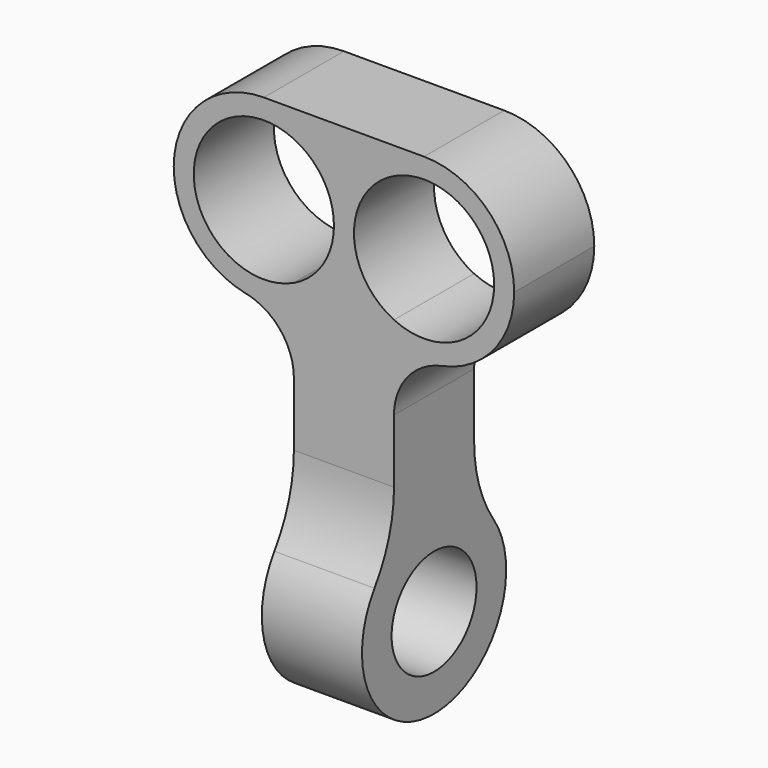
from build123d import *

# Parameters (mm, degrees)
F0_W        = 5
F0_H        = 16
F1_DEPTH    = 5
F2_R        = 4.49999
F3_T1_DEPTH = 22.5
F4_R        = 3
F5_R        = 4.5
F6_DEPTH    = 2.5
F7_R        = 2.65
F8_DEPTH    = 25
F9_R        = 7


# Not quite as in the source:
# - a fillet or chamfer that OpenCascade refuses, or shapes differently, is made with other operations: its cross-section is extruded or revolved along the edge and cut away or added
# - a fillet or chamfer is up to 0.001 mm smaller than in the source, because OpenCascade refuses the exact size


with BuildPart() as f1:
    # F0 (on Front) → F1 (new body)
    with BuildSketch(Plane.XZ):
        with BuildLine():
            Line((8.5, 12.5), (2.5, 12.5))
            Line((2.5, 12.5), (2.5, 11.1622776602))
            ThreePointArc((2.5, 11.1622776602), (5.8708286934, 10.9580398915), (7.5, 8))
            ThreePointArc((7.5, 8), (5.8708286934, 5.0419601085), (2.5, 4.8377223398))
            Line((2.5, 4.8377223398), (2.5, 3.5))
            Line((2.5, 3.5), (8.5, 3.5))
            Line((8.5, 3.5), (8.5, 12.5))
        make_face()
        with BuildLine():
            Line((-2.5, 11.1622776602), (-2.5, 12.5))
            Line((-2.5, 12.5), (-8.5, 12.5))
            Line((-8.5, 12.5), (-8.5, 3.5))
            Line((-8.5, 3.5), (-2.5, 3.5))
            Line((-2.5, 3.5), (-2.5, 4.8377223398))
            ThreePointArc((-2.5, 4.8377223398), (-7.5, 8), (-2.5, 11.1622776602))
        make_face()
        with BuildLine():
            Line((2.5, 11.1622776602), (2.5, 12.5))
            Line((2.5, 12.5), (-2.5, 12.5))
            Line((-2.5, 12.5), (-2.5, 11.1622776602))
            ThreePointArc((-2.5, 11.1622776602), (-1.0419601085, 9.8708286934), (-0.5, 8))
            ThreePointArc((-0.5, 8), (-1.0419601085, 6.1291713066), (-2.5, 4.8377223398))
            Line((-2.5, 4.8377223398), (-2.5, 3.5))
            Line((-2.5, 3.5), (2.5, 3.5))
            Line((2.5, 3.5), (2.5, 4.8377223398))
            ThreePointArc((2.5, 4.8377223398), (0.5, 8), (2.5, 11.1622776602))
        make_face()
        with Locations((0, -4.5)):
            Rectangle(F0_W, F0_H)
    extrude(amount=F1_DEPTH)

    # F2 (radius 4.5 in the source; OpenCascade refuses exactly that, so slightly less here)
    f2_edges = [f1.edges().sort_by_distance(p)[0] for p in [
        (8.5, -2.5, 12.5),
        (-8.5, -2.5, 12.5),
        (8.5, -2.5, 3.5),
        (-8.5, -2.5, 3.5),
    ]]
    fillet(f2_edges, radius=F2_R)

    # F3: fillet of radius 3.5 on 2 edges, made by hand

    # F3_s2 → F3_t1 (cut)
    with BuildSketch(Plane.YZ.offset(-11.25)):
        with BuildLine():
            ThreePointArc((0, -9), (-1.0251262658, -11.4748737342), (-3.5, -12.5))
            Line((-3.5, -12.5), (0, -12.5))
            Line((0, -12.5), (0, -9))
        make_face()
        with BuildLine():
            ThreePointArc((-5, -9), (-3.9748737342, -11.4748737342), (-1.5, -12.5))
            Line((-1.5, -12.5), (-5, -12.5))
            Line((-5, -12.5), (-5, -9))
        make_face()
    extrude(amount=F3_T1_DEPTH, mode=Mode.SUBTRACT)

    # F4
    f4_edges = [f1.edges().sort_by_distance(p)[0] for p in [
        (2.5, -2.5, 3.5),
        (-2.5, -2.5, 3.5),
    ]]
    fillet(f4_edges, radius=F4_R)

    # F5 (on Right) → F6 (join, symmetric)
    with BuildSketch(Plane.YZ):
        with Locations((-2.5, -9)):
            Circle(F5_R)
    extrude(amount=F6_DEPTH, both=True)

    # F7 (on face) → F8 (cut)
    with BuildSketch(Plane.YZ.offset(2.5)):
        with Locations((-2.5, -9)):
            Circle(F7_R)
    extrude(amount=-F8_DEPTH, mode=Mode.SUBTRACT)

    # F9
    f9_edges = [f1.edges().sort_by_distance(p)[0] for p in [
        (0, 0, -5.258343),
        (0, -5, -5.258343),
    ]]
    fillet(f9_edges, radius=F9_R)


solid = f1.part
